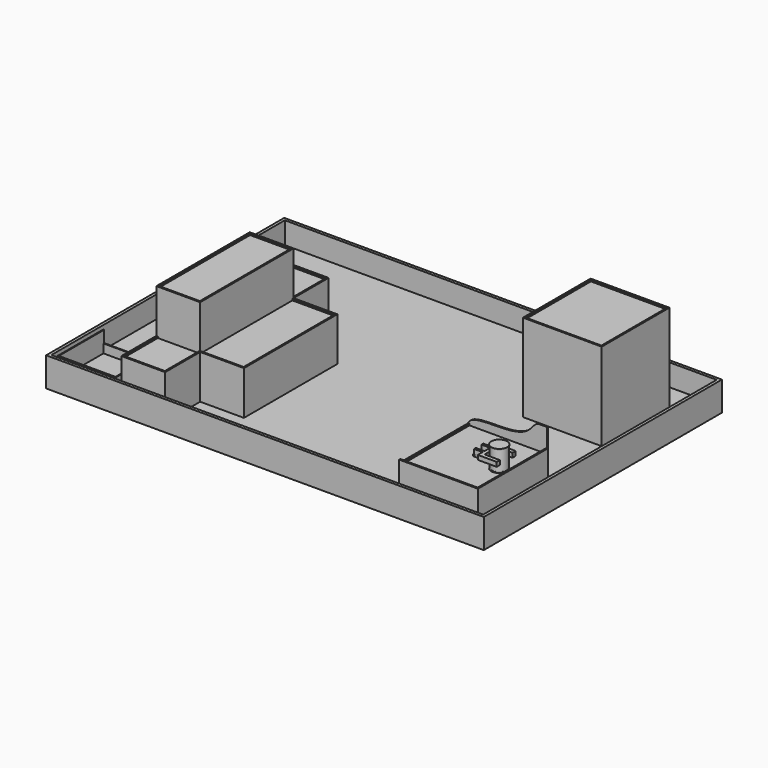
from build123d import *

# Parameters (mm, degrees)
F0_R      = 27.2
F1_DEPTH  = 2.83
F2_R      = 26.4
F3_DEPTH  = 67.36
F4_R      = 27.2
F5_DEPTH  = 2.83
F9_W      = 270
F9_H      = 300
F10_DEPTH = 72
F12_DEPTH = 15
F14_DEPTH = 5
F15_W     = 5
F15_H     = 290
F16_DEPTH = 5
F17_W     = 1500
F17_H     = 1020
F18_DEPTH = 25
F19_W     = 270
F19_H     = 290
F20_DEPTH = 300
F21_W     = 260
F21_H     = 280
F22_DEPTH = 5
F23_W     = 1500
F23_H     = 1020
F23_W_2   = 1480
F23_H_2   = 1000
F24_DEPTH = 75
F26_DEPTH = 150
F27_W     = 150
F27_H     = 400
F28_DEPTH = 150
F29_W     = 140
F29_H     = 390
F30_DEPTH = 5
F31_W     = 140
F31_H     = 145
F31_W_2   = 145
F31_H_2   = 390
F32_DEPTH = 5
F33_R     = 3
F34_DEPTH = 4
F35_R     = 3.99999
F35_2_R   = 3.99999
F36_R     = 3
F37_DEPTH = 8
F38_R     = 3
F39_DEPTH = 8
F40_R     = 3
F40_R_2   = 2.5
F41_DEPTH = 3
F42_R     = 3
F42_R_2   = 2.5
F43_DEPTH = 3
F45_DEPTH = 270.001
F46_W     = 200
F46_H     = 200
F46_W_2   = 194
F46_H_2   = 191
F47_DEPTH = 30
F49_DEPTH = 40
F50_R     = 2.5
F51_DEPTH = 15


# Not quite as in the source:
# - a fillet or chamfer is up to 0.001 mm smaller than in the source, because OpenCascade refuses the exact size
# - a feature names something its author has since deleted; it is built from what else it names


with BuildPart() as f1:
    # F0 (on Top) → F1 (new body)
    with BuildSketch(Plane.XY):
        Circle(F0_R)
    extrude(amount=F1_DEPTH)

    # F2 (on face) → F3 (join)
    with BuildSketch(Plane.XY.offset(2.83)):
        Circle(F2_R)
    extrude(amount=F3_DEPTH)

    # F4 (on face) → F5 (join)
    with BuildSketch(Plane.XY.offset(70.19)):
        Circle(F4_R)
    extrude(amount=F5_DEPTH)


with BuildPart() as f10:
    # F9 (on Top) → F10 (new body)
    with BuildSketch(Plane.XY):
        with Locations((-87.8, 0)):
            Rectangle(F9_W, F9_H)
    extrude(amount=-F10_DEPTH)

    # F11 (on face) → F12 (join)
    with BuildSketch(Plane.XY):
        Polygon((-222.8, -145), (-222.8, -150), (47.2, -150), (47.2, 150), (42.2, 150), (42.2, -145), align=None)
    extrude(amount=F12_DEPTH)

    # F13 (on face) → F14 (join)
    with BuildSketch(Plane(origin=(0, 150, 0), x_dir=(-1, 0, 0), z_dir=(0, 1, 0))):
        with BuildLine():
            Line((-21.3134280931, 81.3575685024), (-47.2, 81.3575685024))
            Line((-47.2, 81.3575685024), (-47.2, -72))
            Line((-47.2, -72), (222.8, -72))
            Line((222.8, -72), (222.8, 0))
            add(Edge.make_bspline(
                [(-21.3134280931, 81.3575685024), (-6.3059147253, 81.3822787863), (12.9585432644, 38.1268753575), (103.6097013063, 23.6068887567), (223.0224295336, 30.7718731823), (222.8, 0)],
                knots=[0, 0, 0, 0, 0.2487100673, 0.6151112321, 1, 1, 1, 1], degree=3))
        make_face()
    extrude(amount=-F14_DEPTH)

    # F15 (on face) → F16 (join)
    with BuildSketch(Plane.XY):
        with Locations((-220.3, 0)):
            Rectangle(F15_W, F15_H)
    extrude(amount=F16_DEPTH)

    # F17 (on face) → F18 (join)
    with BuildSketch(Plane(origin=(0, 0, -72), x_dir=(1, 0, 0), z_dir=(0, 0, -1))):
        with Locations((-602.8, -260)):
            Rectangle(F17_W, F17_H)
    extrude(amount=F18_DEPTH)

    # F19 (on face) → F20 (join)
    with BuildSketch(Plane.XY.offset(-72)):
        with Locations((-87.8, 525)):
            Rectangle(F19_W, F19_H)
    extrude(amount=F20_DEPTH)

    # F21 (on face) → F22 (cut)
    with BuildSketch(Plane.XY.offset(228)):
        with Locations((-87.8, 525)):
            Rectangle(F21_W, F21_H)
    extrude(amount=-F22_DEPTH, mode=Mode.SUBTRACT)

    # F23 (on face) → F24 (join)
    with BuildSketch(Plane.XY.offset(-72)):
        with Locations((-602.8, 260)):
            Rectangle(F23_W, F23_H)
        with Locations((-602.8, 260)):
            Rectangle(F23_W_2, F23_H_2, mode=Mode.SUBTRACT)
    extrude(amount=F24_DEPTH)

    # F25 (on face) → F26 (join)
    with BuildSketch(Plane.XY.offset(-72)):
        Polygon((-952.8, 460), (-1102.8, 460), (-1102.8, -240), (-952.8, -240), (-952.8, -90), (-802.8, -90), (-802.8, 310), (-952.8, 310), align=None)
    extrude(amount=F26_DEPTH)

    # F27 (on face) → F28 (join)
    with BuildSketch(Plane.XY.offset(78)):
        with Locations((-1027.8, 110)):
            Rectangle(F27_W, F27_H)
    extrude(amount=F28_DEPTH)

    # F29 (on face) → F30 (cut)
    with BuildSketch(Plane.XY.offset(228)):
        with Locations((-1027.8, 110)):
            Rectangle(F29_W, F29_H)
    extrude(amount=-F30_DEPTH, mode=Mode.SUBTRACT)

    # F31 (on face) → F32 (cut)
    with BuildSketch(Plane.XY.offset(78)):
        with Locations((-1027.8, 382.5)):
            Rectangle(F31_W, F31_H)
        with Locations((-880.3, 110)):
            Rectangle(F31_W_2, F31_H_2)
        with Locations((-1027.8, -162.5)):
            Rectangle(F31_W, F31_H)
    extrude(amount=-F32_DEPTH, mode=Mode.SUBTRACT)

    # F46 (on face) → F47 (join)
    with BuildSketch(Plane.XY.offset(-72)):
        with Locations((-1232.8, -130)):
            Rectangle(F46_W, F46_H)
        with Locations((-1232.8, -128.5)):
            Rectangle(F46_W_2, F46_H_2, mode=Mode.SUBTRACT)
    extrude(amount=F47_DEPTH)

    # F48 (on face) → F49 (join)
    with BuildSketch(Plane.XY.offset(-42)):
        Polygon((-1329.8, -30), (-1332.8, -30), (-1332.8, -230), (-1329.8, -230), (-1135.8, -230), (-1132.8, -230), (-1132.8, -30), (-1135.8, -30), (-1135.8, -224), (-1329.8, -224), align=None)
    extrude(amount=F49_DEPTH)


with BuildPart() as f34:
    # F33 (on offset) → F34 (new body, symmetric)
    with BuildSketch(Plane.XY.offset(25)):
        with BuildLine():
            Line((-55, -12), (-74.5, -12))
            Line((-74.5, -12), (-74.5, -13))
            Line((-74.5, -13), (-65.6457513111, -13))
            ThreePointArc((-65.6457513111, -13), (-67, -16), (-65.6457513111, -19))
            Line((-65.6457513111, -19), (-74.5, -19))
            Line((-74.5, -19), (-74.5, -20))
            Line((-74.5, -20), (-55, -20))
            ThreePointArc((-55, -20), (-51, -16), (-55, -12))
        make_face()
        with Locations((-63, -16)):
            Circle(F33_R, mode=Mode.SUBTRACT)
        with Locations((-55, -16)):
            Circle(F33_R, mode=Mode.SUBTRACT)
    extrude(amount=F34_DEPTH, both=True)

    # F35 (radius 4 in the source; OpenCascade refuses exactly that, so slightly less here)
    f35_edges = [f34.edges().sort_by_distance(p)[0] for p in [
        (-74.5, -19.5, 29),
        (-74.5, -12.5, 29),
        (-74.5, -19.5, 21),
        (-74.5, -12.5, 21),
    ]]
    fillet(f35_edges, radius=F35_R)

    # F36 (on face) → F37 (join, through all)
    with BuildSketch(Plane.XZ.offset(20)):
        with Locations((-70.5, 25)):
            Circle(F36_R)
    extrude(amount=-F37_DEPTH)

    # F42 (on offset) → F43 (join, symmetric)
    with BuildSketch(Plane.XY.offset(25)):
        with Locations((-63, -16)):
            Circle(F42_R)
        with Locations((-63, -16)):
            Circle(F42_R_2, mode=Mode.SUBTRACT)
        with Locations((-55, -16)):
            Circle(F42_R)
        with Locations((-55, -16)):
            Circle(F42_R_2, mode=Mode.SUBTRACT)
    extrude(amount=F43_DEPTH, both=True)


with BuildPart() as f34b:
    # F33 (on offset) → F34, piece 2 (new body, symmetric)
    with BuildSketch(Plane.XY.offset(25)):
        with BuildLine():
            Line((-74.5, 13), (-74.5, 12))
            Line((-74.5, 12), (-55, 12))
            ThreePointArc((-55, 12), (-51, 16), (-55, 20))
            Line((-55, 20), (-74.5, 20))
            Line((-74.5, 20), (-74.5, 19))
            Line((-74.5, 19), (-65.6457513111, 19))
            ThreePointArc((-65.6457513111, 19), (-67, 16), (-65.6457513111, 13))
            Line((-65.6457513111, 13), (-74.5, 13))
        make_face()
        with Locations((-63, 16)):
            Circle(F33_R, mode=Mode.SUBTRACT)
        with Locations((-55, 16)):
            Circle(F33_R, mode=Mode.SUBTRACT)
    extrude(amount=F34_DEPTH, both=True)

    # F35#2 (radius 4 in the source; OpenCascade refuses exactly that, so slightly less here)
    f35_2_edges = [f34b.edges().sort_by_distance(p)[0] for p in [
        (-74.5, 12.5, 29),
        (-74.5, 19.5, 29),
        (-74.5, 19.5, 21),
        (-74.5, 12.5, 21),
    ]]
    fillet(f35_2_edges, radius=F35_2_R)

    # F38 (on face) → F39 (join, through all)
    with BuildSketch(Plane(origin=(0, 20, 0), x_dir=(-1, 0, 0), z_dir=(0, 1, 0))):
        with Locations((70.5, 25)):
            Circle(F38_R)
    extrude(amount=-F39_DEPTH)

    # F40 (on offset) → F41 (join, symmetric)
    with BuildSketch(Plane.XY.offset(25)):
        with Locations((-55, 16)):
            Circle(F40_R)
        with Locations((-55, 16)):
            Circle(F40_R_2, mode=Mode.SUBTRACT)
        with Locations((-63, 16)):
            Circle(F40_R)
        with Locations((-63, 16)):
            Circle(F40_R_2, mode=Mode.SUBTRACT)
    extrude(amount=F41_DEPTH, both=True)


with BuildPart() as f45_tool:
    # F44 (on face) → F45 (new body, through all)
    with BuildSketch(Plane(origin=(0, 20, 0), x_dir=(-1, 0, 0), z_dir=(0, 1, 0))):
        with BuildLine():
            Line((71.5, 26), (71.5, 27.2912878475))
            ThreePointArc((71.5, 27.2912878475), (70.5, 27.5), (69.5, 27.2912878475))
            Line((69.5, 27.2912878475), (69.5, 26))
            Line((69.5, 26), (68.2087121525, 26))
            ThreePointArc((68.2087121525, 26), (68, 25), (68.2087121525, 24))
            Line((68.2087121525, 24), (69.5, 24))
            Line((69.5, 24), (69.5, 22.7087121525))
            ThreePointArc((69.5, 22.7087121525), (70.5, 22.5), (71.5, 22.7087121525))
            Line((71.5, 22.7087121525), (71.5, 24))
            Line((71.5, 24), (72.7912878475, 24))
            ThreePointArc((72.7912878475, 24), (73, 25), (72.7912878475, 26))
            Line((72.7912878475, 26), (71.5, 26))
        make_face()
    extrude(amount=-F45_DEPTH)


with BuildPart() as f34_1:
    add(f34.part)

    # F45: cut by f45_tool
    add(f45_tool.part, mode=Mode.SUBTRACT)


with BuildPart() as f34b_1:
    add(f34b.part)

    # F45: cut by f45_tool
    add(f45_tool.part, mode=Mode.SUBTRACT)


with BuildPart() as f51:
    # F50 (on face) → F51 (new body)
    with BuildSketch(Plane.XY.offset(29)):
        Polygon((-70.5, 20), (-70.5, 12), (-40.7567732036, 12), (-40.7567732036, -12.0408376679), (-70.5, -12.0408376679), (-70.5, -20.1567281038), (-40.7567732036, -20.1567281038), (-40.7567732036, -40.5738651752), (24.02815409, -40.5738651752), (24.02815409, -27.129650116), (-28.3627118915, -27.129650116), (-28.3627118915, 27.129650116), (24.02815409, 27.129650116), (24.02815409, 40.5738651752), (-40.7567732036, 40.5738651752), (-40.7567732036, 20), align=None)
        with Locations((-63, -16)):
            Circle(F50_R, mode=Mode.SUBTRACT)
        with Locations((-55, -16)):
            Circle(F50_R, mode=Mode.SUBTRACT)
        with Locations((-63, 16)):
            Circle(F50_R, mode=Mode.SUBTRACT)
        with Locations((-55, 16)):
            Circle(F50_R, mode=Mode.SUBTRACT)
    extrude(amount=F51_DEPTH)


solid = Compound([f1.part, f10.part, f34_1.part, f34b_1.part, f51.part])
